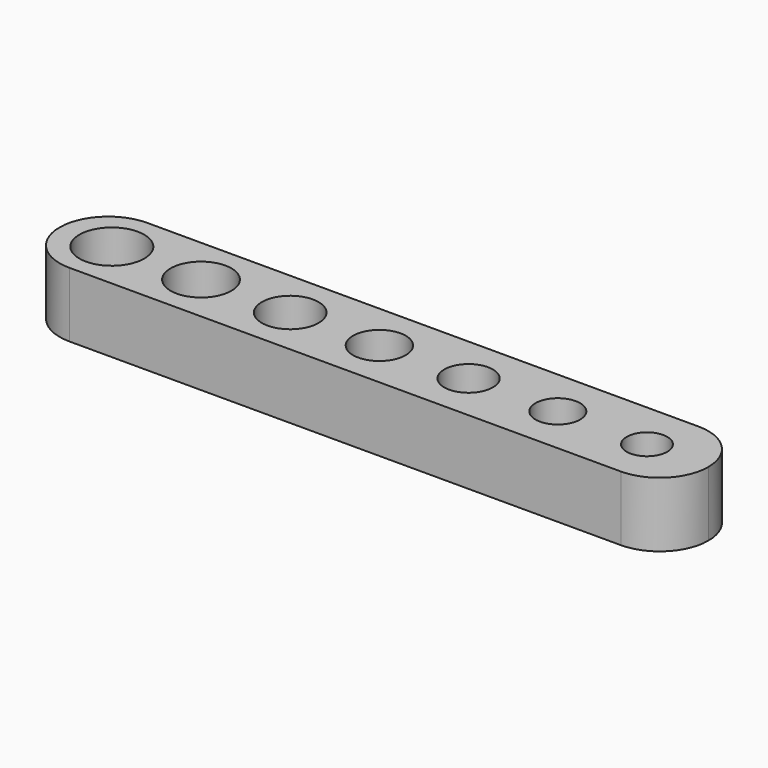
from build123d import *

# Parameters (mm, degrees)
F0_W     = 40
F0_H     = 6
F0_R     = 2
F0_R_2   = 1.875
F0_R_3   = 1.75
F0_R_4   = 1.625
F0_R_5   = 1.5
F0_R_6   = 1.375
F0_R_7   = 1.25
F1_DEPTH = 4
F2_R     = 2.99999


# Not quite as in the source:
# - a fillet or chamfer is up to 0.001 mm smaller than in the source, because OpenCascade refuses the exact size


with BuildPart() as f1:
    # F0 (on Top) → F1 (new body)
    with BuildSketch(Plane.XY):
        with Locations((-20, 3)):
            Rectangle(F0_W, F0_H)
        with Locations((-36.7836877704, 3)):
            Circle(F0_R, mode=Mode.SUBTRACT)
        with Locations((-31.2836877704, 3)):
            Circle(F0_R_2, mode=Mode.SUBTRACT)
        with Locations((-25.7836877704, 3)):
            Circle(F0_R_3, mode=Mode.SUBTRACT)
        with Locations((-20.2836877704, 3)):
            Circle(F0_R_4, mode=Mode.SUBTRACT)
        with Locations((-14.7836877704, 3)):
            Circle(F0_R_5, mode=Mode.SUBTRACT)
        with Locations((-9.2836877704, 3)):
            Circle(F0_R_6, mode=Mode.SUBTRACT)
        with Locations((-3.7836877704, 3)):
            Circle(F0_R_7, mode=Mode.SUBTRACT)
    extrude(amount=F1_DEPTH)

    # F2 (radius 3 in the source; OpenCascade refuses exactly that, so slightly less here)
    f2_edges = [f1.edges().sort_by_distance(p)[0] for p in [
        (0, 0, 2),
        (0, 6, 2),
        (-40, 0, 2),
        (-40, 6, 2),
    ]]
    fillet(f2_edges, radius=F2_R)


solid = f1.part
